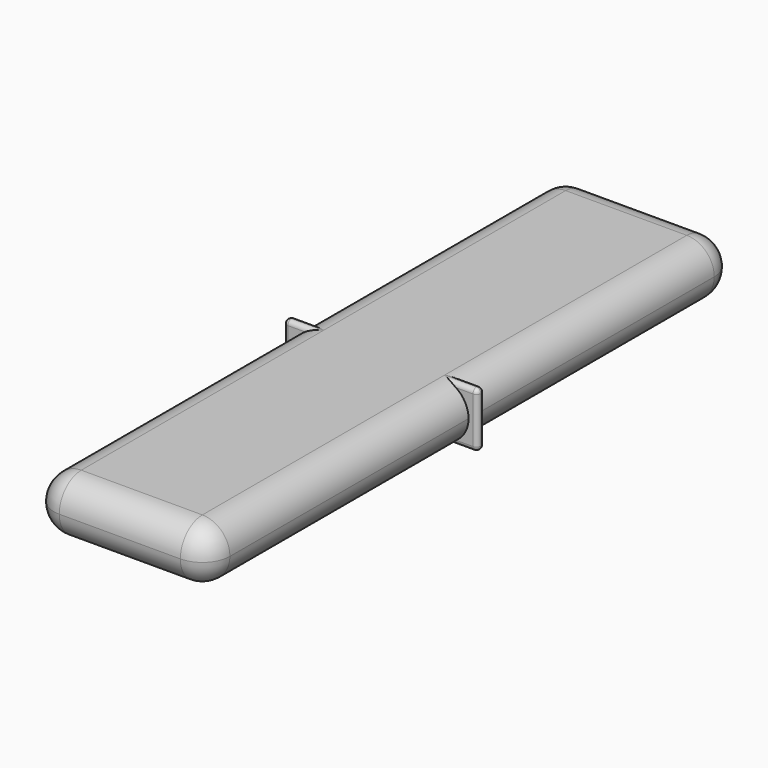
from build123d import *

# Parameters (mm, degrees)
F1_DEPTH = 6.35
F2_R     = 0.50799
F3_F1_R  = 3.175
F3_F2_R  = 3.175
F3_F3_R  = 3.175
F3_F4_R  = 3.175
F3_F5_R  = 3.175
F3_F6_R  = 3.175
F3_F7_R  = 3.1746
F3_F8_R  = 3.1746
F4_R     = 7.62
F5_DEPTH = 2.54


# Not quite as in the source:
# - a fillet or chamfer is up to 0.001 mm smaller than in the source, because OpenCascade refuses the exact size


with BuildPart() as f1:
    # F0 (on Top) → F1 (new body)
    with BuildSketch(Plane.XY):
        Polygon((0, 7.7513456765), (0, 45.3433456765), (-20.32, 45.3433456765), (-20.32, 7.7513456765), (-21.336, 7.7513456765), (-21.336, 6.7353456765), (-20.32, 6.7353456765), (-20.32, -30.8566543235), (0, -30.8566543235), (0, 6.7353456765), (1.016, 6.7353456765), (1.016, 7.7513456765), align=None)
    extrude(amount=F1_DEPTH)

    # F2 (radius 0.508 in the source; OpenCascade refuses exactly that, so slightly less here)
    f2_edges = [f1.edges().sort_by_distance(p)[0] for p in [
        (1.016, 6.735346, 3.175),
        (1.016, 7.751346, 3.175),
        (1.016, 7.243346, 0),
        (1.016, 7.243346, 6.35),
        (0.508, 7.751346, 6.35),
        (0.508, 6.735346, 6.35),
        (0.508, 6.735346, 0),
        (0.508, 7.751346, 0),
        (-21.336, 7.751346, 3.175),
        (-21.336, 6.735346, 3.175),
        (-21.336, 7.243346, 0),
        (-21.336, 7.243346, 6.35),
        (-20.828, 7.751346, 6.35),
        (-20.828, 6.735346, 6.35),
        (-20.828, 7.751346, 0),
        (-20.828, 6.735346, 0),
    ]]
    fillet(f2_edges, radius=F2_R)

    # F3: fillet of radius 3.175 on 16 edges, made by hand

    # F3_f1
    f3_f1_edges = [f1.edges().sort_by_distance(p)[0] for p in [
        (0, -30.8566543235, 3.175),
    ]]
    fillet(f3_f1_edges, radius=F3_F1_R)

    # F3_f2
    f3_f2_edges = [f1.edges().sort_by_distance(p)[0] for p in [
        (-20.32, -30.8566543235, 3.175),
    ]]
    fillet(f3_f2_edges, radius=F3_F2_R)

    # F3_f3
    f3_f3_edges = [f1.edges().sort_by_distance(p)[0] for p in [
        (0, 45.3433456765, 3.175),
    ]]
    fillet(f3_f3_edges, radius=F3_F3_R)

    # F3_f4
    f3_f4_edges = [f1.edges().sort_by_distance(p)[0] for p in [
        (-20.32, 45.3433456765, 3.175),
    ]]
    fillet(f3_f4_edges, radius=F3_F4_R)

    # F3_f5
    f3_f5_edges = [f1.edges().sort_by_distance(p)[0] for p in [
        (-10.16, -30.8566543235, 0),
    ]]
    fillet(f3_f5_edges, radius=F3_F5_R)

    # F3_f6
    f3_f6_edges = [f1.edges().sort_by_distance(p)[0] for p in [
        (-10.16, 45.3433456765, 0),
    ]]
    fillet(f3_f6_edges, radius=F3_F6_R)

    # F3_f7 (radius 3.175 in the source; OpenCascade refuses exactly that, so slightly less here)
    f3_f7_edges = [f1.edges().sort_by_distance(p)[0] for p in [
        (-10.16, 45.3433456765, 6.35),
    ]]
    fillet(f3_f7_edges, radius=F3_F7_R)

    # F3_f8 (radius 3.175 in the source; OpenCascade refuses exactly that, so slightly less here)
    f3_f8_edges = [f1.edges().sort_by_distance(p)[0] for p in [
        (-10.16, -30.8566543235, 6.35),
    ]]
    fillet(f3_f8_edges, radius=F3_F8_R)

    # F4 (on face) → F5 (cut)
    with BuildSketch(Plane(origin=(0, 0, 0), x_dir=(1, 0, 0), z_dir=(0, 0, -1))):
        with Locations((-10.16, -7.2433456765)):
            Circle(F4_R)
    extrude(amount=-F5_DEPTH, mode=Mode.SUBTRACT)


solid = f1.part
